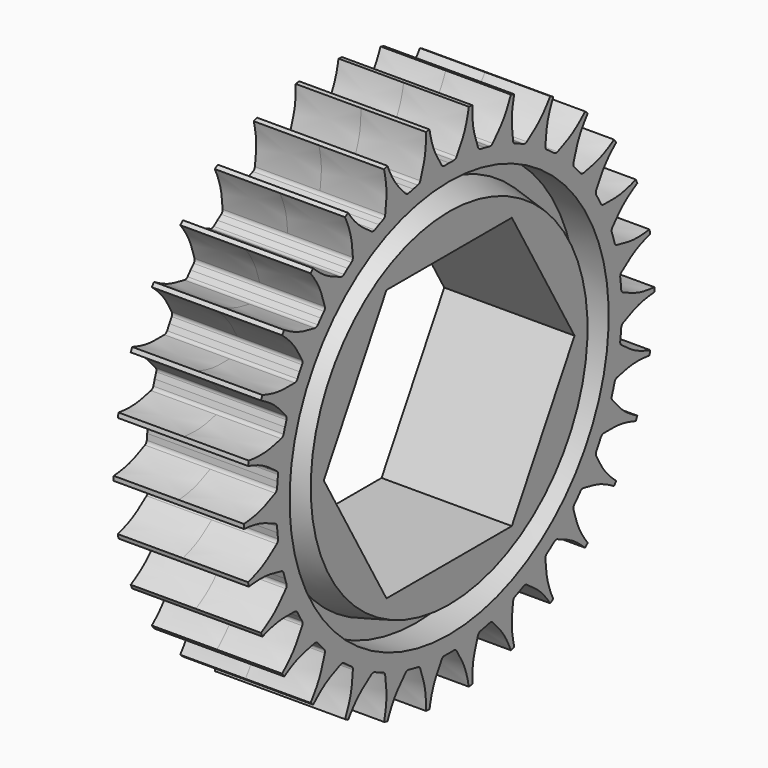
from build123d import *

# Parameters (mm, degrees)
F3_DEPTH        = 8.001
F5_DEPTH        = 4
F5_COPIES_COUNT = 30


# Not quite as in the source:
# - ends of sketch curves that miss each other by under 0.0002 mm in the source are joined
# - a feature of the source that left no trace in its solid (it failed there, or was rolled back) is left out
# - a pattern or mirror of a feature is missing from the dataset's text; its kind, count and spacing are read off the source's solid


with BuildPart() as f1:
    # F0 (on Front) → F1 (revolve)
    with BuildSketch(Plane.XZ):
        Polygon((4, 15.75), (0, 15.75), (-4, 15.75), (-4, 12.25), (-2, 12.25), (-2, 11.125), (-4, 10.625), (-4, 9.625), (0, 9.625), (4, 9.625), (4, 10.625), (2, 11.125), (2, 12.25), (4, 12.25), align=None)
        Polygon((0, 9.625), (-4, 9.625), (-4, 0), (4, 0), (4, 9.625), align=None)
    revolve(axis=Axis((0, 0, 0), (-1, 0, 0)))

    # F2 (on face) → F3 (cut, through all)
    with BuildSketch(Plane(origin=(-4, 0, 0), x_dir=(0, -1, 0), z_dir=(-1, 0, 0))):
        Polygon((4.8125, 8.3354945114), (-4.8125, 8.3354945114), (-9.625, 0), (-4.8125, -8.3354945114), (4.8125, -8.3354945114), (9.625, 0), align=None)
    extrude(amount=-F3_DEPTH, mode=Mode.SUBTRACT)

    # F4 (on Right) → F5 (cut, symmetric)
    with BuildSketch(Plane.YZ):
        with BuildLine():
            ThreePointArc((0.3577630421, 13.2432485521), (0.4820536544, 13.2736495516), (0.5750030657, 13.3615858013))
            add(Edge.make_bspline(
                [(0.5750030657, 13.3615858013), (0.8087766949, 13.7393080208), (1.269265933, 14.5098524547), (1.4423170655, 15.3283085169), (1.5189511469, 15.7252904028)],
                knots=[0.0499106914, 0.0499106914, 0.0499106914, 0.0499106914, 0.5171376294, 1, 1, 1, 1], degree=3))
            Line((1.5189511469, 15.7252904028), (0, 15.7816819847))
            Line((0, 15.7816819847), (-1.5189511469, 15.7252904028))
            add(Edge.make_bspline(
                [(-0.575003065, 13.3615858002), (-0.8087766945, 13.7393080201), (-1.2692659329, 14.5098524543), (-1.4423170655, 15.3283085169), (-1.5189511469, 15.7252904028)],
                knots=[0.049910691, 0.049910691, 0.049910691, 0.049910691, 0.5171376294, 1, 1, 1, 1], degree=3))
            ThreePointArc((-0.575003065, 13.3615858002), (-0.4820541764, 13.2736544596), (-0.3577630421, 13.2432485521))
            Line((-0.3577630421, 13.2432485521), (0, 13.25))
            Line((0, 13.25), (0.3577630421, 13.2432485521))
        make_face()
    f5 = extrude(amount=F5_DEPTH, both=True, mode=Mode.SUBTRACT)

    # F5_copies: F5 ×30 about axis
    f5_copies_axis = Axis((0, 0, 0), (1, 0, 0))
    for i in range(1, F5_COPIES_COUNT):
        add(f5.rotate(f5_copies_axis, i * 360 / F5_COPIES_COUNT), mode=Mode.SUBTRACT)


solid = f1.part
